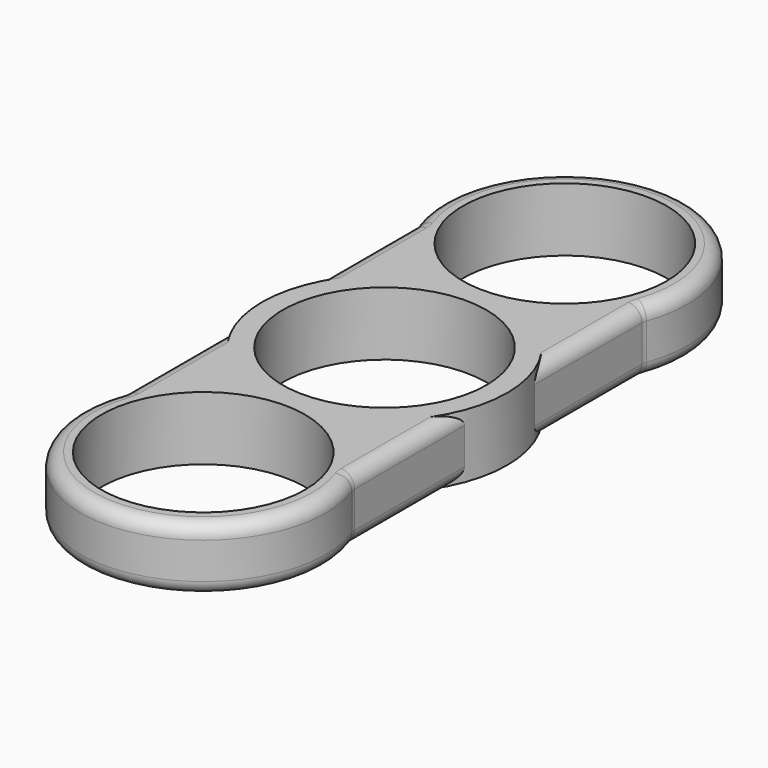
from build123d import *

# Parameters (mm, degrees)
F0_R     = 11.2
F1_DEPTH = 7
F2_F1_R  = 1.5
F2_F2_R  = 1.5


with BuildPart() as f1:
    # F0 (on Top) → F1 (new body)
    with BuildSketch(Plane.XY):
        with BuildLine():
            Line((-12.5890504837, 19.9107848701), (-12.5890504837, 4.8750187608))
            ThreePointArc((-12.5890504837, 4.8750187608), (-13.4998898549, 0.0545335167), (-12.6280247824, -4.773153056))
            Line((-12.6280247824, -4.773153056), (-12.6280247824, -20.1613976912))
            ThreePointArc((-12.6280247824, -20.1613976912), (0, -38.4345507473), (12.6280247824, -20.1613976912))
            Line((12.6280247824, -20.1613976912), (12.6280247824, -4.773153056))
            ThreePointArc((12.6280247824, -4.773153056), (13.4998898549, 0.0545335167), (12.5890504837, 4.8750187608))
            Line((12.5890504837, 4.8750187608), (12.5890504837, 19.9107848701))
            ThreePointArc((12.5890504837, 19.9107848701), (0, 38.2858036309), (-12.5890504837, 19.9107848701))
        make_face()
        with Locations((0, -24.9345507473)):
            Circle(F0_R, mode=Mode.SUBTRACT)
        Circle(F0_R, mode=Mode.SUBTRACT)
        with Locations((0, 24.7858036309)):
            Circle(F0_R, mode=Mode.SUBTRACT)
    extrude(amount=F1_DEPTH)

    # F2: fillet of radius 1.5 on 8 edges, made by hand

    # F2_f1
    f2_f1_edges = [f1.edges().sort_by_distance(p)[0] for p in [
        (12.5890504837, 19.9107848701, 3.5),
        (-12.5890504837, 19.9107848701, 3.5),
        (-12.6280247824, -20.1613976912, 3.5),
        (12.6280247824, -20.1613976912, 3.5),
    ]]
    fillet(f2_f1_edges, radius=F2_F1_R)

    # F2_f2
    f2_f2_edges = [f1.edges().sort_by_distance(p)[0] for p in [
        (0, 38.2858036309, 0),
        (0, 38.2858036309, 7),
        (0, -38.4345507473, 0),
        (0, -38.4345507473, 7),
        (-12.6499849119, -20.1505476521, 7),
        (12.6499849119, -20.1505476521, 7),
        (-12.6499849119, -20.1505476521, 0),
        (12.6499849119, -20.1505476521, 0),
        (12.6119997783, 19.8995023273, 7),
        (-12.6119997783, 19.8995023273, 7),
        (12.6119997783, 19.8995023273, 0),
        (-12.6119997783, 19.8995023273, 0),
    ]]
    fillet(f2_f2_edges, radius=F2_F2_R)


solid = f1.part
